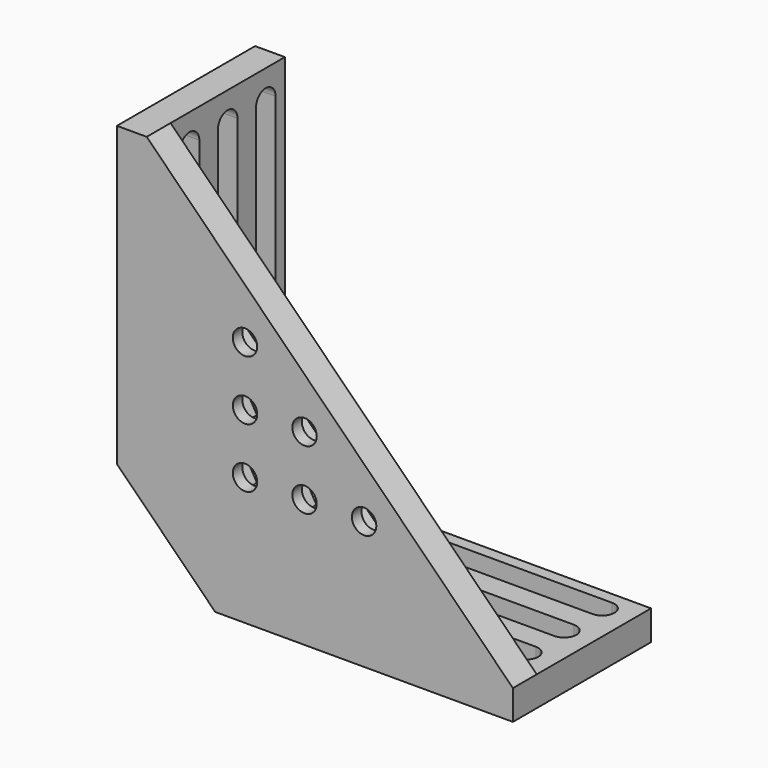
from build123d import *

# Parameters (mm, degrees)
F1_DEPTH = 5
F3_ANGLE = 90
F7_R     = 2.05
F8_DEPTH = 5
F9_DEPTH = 3


# Not quite as in the source:
# - a feature names something its author has since deleted; it is built from what else it names


with BuildPart() as f1:
    # F0 (on Top) → F1 (new body)
    with BuildSketch(Plane.XY):
        Polygon((29, 12), (-21, 12), (-21, -12), (0, -12), (29, -12), align=None)
        with BuildLine():
            ThreePointArc((-16, -10.05), (-18.05, -8), (-16, -5.95))
            Line((-16, -5.95), (0, -5.95))
            Line((0, -5.95), (24, -5.95))
            ThreePointArc((24, -5.95), (26.05, -8), (24, -10.05))
            Line((24, -10.05), (0, -10.05))
            Line((0, -10.05), (-16, -10.05))
        make_face(mode=Mode.SUBTRACT)
        with BuildLine():
            Line((0, -2.05), (-16, -2.05))
            ThreePointArc((-16, -2.05), (-18.05, 0), (-16, 2.05))
            Line((-16, 2.05), (0, 2.05))
            Line((0, 2.05), (24, 2.05))
            ThreePointArc((24, 2.05), (26.05, 0), (24, -2.05))
            Line((24, -2.05), (0, -2.05))
        make_face(mode=Mode.SUBTRACT)
        with BuildLine():
            Line((24, 5.95), (0, 5.95))
            Line((0, 5.95), (-16, 5.95))
            ThreePointArc((-16, 5.95), (-18.05, 8), (-16, 10.05))
            Line((-16, 10.05), (0, 10.05))
            Line((0, 10.05), (24, 10.05))
            ThreePointArc((24, 10.05), (26.05, 8), (24, 5.95))
        make_face(mode=Mode.SUBTRACT)
    extrude(amount=F1_DEPTH)


with BuildPart() as f3_1:
    # F3: copy of F1
    add(f1.part.rotate(Axis((-21, 0, 2.5), (0, -1, 0)), F3_ANGLE))


with BuildPart() as f3_1_1:
    # F4: moved
    add(f3_1.part.moved(Location((0, 0, 14))))


with BuildPart() as f3_1_2:
    # F5: moved
    add(f3_1_1.part.moved(Location((-14, 0, 0))))


with BuildPart() as f1_1:
    add(f1.part)

    add(f3_1_2.part)  # F8 merges F3_1
    # F7 (on 3pt) → F8 (join)
    with BuildSketch(Plane.XZ.offset(12)):
        Polygon((-37.5, 16.5), (-21, 0), (29, 0), (29, 5), (-32.5, 66.5), (-37.5, 66.5), align=None)
        Polygon((-19.9926406871, 21.5073593129), (-17.9926406871, 24.971460928), (-13.9926406871, 24.971460928), (-11.9926406871, 21.5073593129), (-13.9926406871, 18.0432576977), (-17.9926406871, 18.0432576977), align=None, mode=Mode.SUBTRACT)
        Polygon((-9.9926406871, 21.5073593129), (-7.9926406871, 24.971460928), (-3.9926406871, 24.971460928), (-1.9926406871, 21.5073593129), (-3.9926406871, 18.0432576977), (-7.9926406871, 18.0432576977), align=None, mode=Mode.SUBTRACT)
        Polygon((-19.9926406871, 31.5073593129), (-17.9926406871, 34.971460928), (-13.9926406871, 34.971460928), (-11.9926406871, 31.5073593129), (-13.9926406871, 28.0432576977), (-17.9926406871, 28.0432576977), align=None, mode=Mode.SUBTRACT)
        Polygon((-9.8563439923, 30.4720831325), (-8.8210678119, 34.3357864376), (-4.9573645067, 35.371062618), (-2.128937382, 32.5426354933), (-3.1642135624, 28.6789321881), (-7.0279168675, 27.6436560077), align=None, mode=Mode.SUBTRACT)
        Polygon((0.1436560077, 20.4720831325), (1.1789321881, 24.3357864376), (5.0426354933, 25.371062618), (7.871062618, 22.5426354933), (6.8357864376, 18.6789321881), (2.9720831325, 17.6436560077), align=None, mode=Mode.SUBTRACT)
        Polygon((-19.8563439923, 40.4720831325), (-18.8210678119, 44.3357864376), (-14.9573645067, 45.371062618), (-12.128937382, 42.5426354933), (-13.1642135624, 38.6789321881), (-17.0279168675, 37.6436560077), align=None, mode=Mode.SUBTRACT)
        Polygon((-4.9573645067, 35.371062618), (-8.8210678119, 34.3357864376), (-9.8563439923, 30.4720831325), (-7.0279168675, 27.6436560077), (-3.1642135624, 28.6789321881), (-2.128937382, 32.5426354933), align=None)
        with Locations((-5.9926406871, 31.5073593129)):
            Circle(F7_R, mode=Mode.SUBTRACT)
        Polygon((-14.9573645067, 45.371062618), (-18.8210678119, 44.3357864376), (-19.8563439923, 40.4720831325), (-17.0279168675, 37.6436560077), (-13.1642135624, 38.6789321881), (-12.128937382, 42.5426354933), align=None)
        with Locations((-15.9926406871, 41.5073593129)):
            Circle(F7_R, mode=Mode.SUBTRACT)
        Polygon((-13.9926406871, 34.971460928), (-17.9926406871, 34.971460928), (-19.9926406871, 31.5073593129), (-17.9926406871, 28.0432576977), (-13.9926406871, 28.0432576977), (-11.9926406871, 31.5073593129), align=None)
        with Locations((-15.9926406871, 31.5073593129)):
            Circle(F7_R, mode=Mode.SUBTRACT)
        Polygon((-13.9926406871, 24.971460928), (-17.9926406871, 24.971460928), (-19.9926406871, 21.5073593129), (-17.9926406871, 18.0432576977), (-13.9926406871, 18.0432576977), (-11.9926406871, 21.5073593129), align=None)
        with Locations((-15.9926406871, 21.5073593129)):
            Circle(F7_R, mode=Mode.SUBTRACT)
        Polygon((-3.9926406871, 24.971460928), (-7.9926406871, 24.971460928), (-9.9926406871, 21.5073593129), (-7.9926406871, 18.0432576977), (-3.9926406871, 18.0432576977), (-1.9926406871, 21.5073593129), align=None)
        with Locations((-5.9926406871, 21.5073593129)):
            Circle(F7_R, mode=Mode.SUBTRACT)
        Polygon((5.0426354933, 25.371062618), (1.1789321881, 24.3357864376), (0.1436560077, 20.4720831325), (2.9720831325, 17.6436560077), (6.8357864376, 18.6789321881), (7.871062618, 22.5426354933), align=None)
        with Locations((4.0073593129, 21.5073593129)):
            Circle(F7_R, mode=Mode.SUBTRACT)
    extrude(amount=F8_DEPTH)

    # F7 (on 3pt) → F9 (cut)
    with BuildSketch(Plane.XZ.offset(12)):
        Polygon((-4.9573645067, 35.371062618), (-8.8210678119, 34.3357864376), (-9.8563439923, 30.4720831325), (-7.0279168675, 27.6436560077), (-3.1642135624, 28.6789321881), (-2.128937382, 32.5426354933), align=None)
        with Locations((-5.9926406871, 31.5073593129)):
            Circle(F7_R, mode=Mode.SUBTRACT)
        Polygon((5.0426354933, 25.371062618), (1.1789321881, 24.3357864376), (0.1436560077, 20.4720831325), (2.9720831325, 17.6436560077), (6.8357864376, 18.6789321881), (7.871062618, 22.5426354933), align=None)
        with Locations((4.0073593129, 21.5073593129)):
            Circle(F7_R, mode=Mode.SUBTRACT)
        Polygon((-3.9926406871, 24.971460928), (-7.9926406871, 24.971460928), (-9.9926406871, 21.5073593129), (-7.9926406871, 18.0432576977), (-3.9926406871, 18.0432576977), (-1.9926406871, 21.5073593129), align=None)
        with Locations((-5.9926406871, 21.5073593129)):
            Circle(F7_R, mode=Mode.SUBTRACT)
        Polygon((-13.9926406871, 24.971460928), (-17.9926406871, 24.971460928), (-19.9926406871, 21.5073593129), (-17.9926406871, 18.0432576977), (-13.9926406871, 18.0432576977), (-11.9926406871, 21.5073593129), align=None)
        with Locations((-15.9926406871, 21.5073593129)):
            Circle(F7_R, mode=Mode.SUBTRACT)
        Polygon((-13.9926406871, 34.971460928), (-17.9926406871, 34.971460928), (-19.9926406871, 31.5073593129), (-17.9926406871, 28.0432576977), (-13.9926406871, 28.0432576977), (-11.9926406871, 31.5073593129), align=None)
        with Locations((-15.9926406871, 31.5073593129)):
            Circle(F7_R, mode=Mode.SUBTRACT)
        Polygon((-14.9573645067, 45.371062618), (-18.8210678119, 44.3357864376), (-19.8563439923, 40.4720831325), (-17.0279168675, 37.6436560077), (-13.1642135624, 38.6789321881), (-12.128937382, 42.5426354933), align=None)
        with Locations((-15.9926406871, 41.5073593129)):
            Circle(F7_R, mode=Mode.SUBTRACT)
    extrude(amount=F9_DEPTH, mode=Mode.SUBTRACT)


solid = f1_1.part
